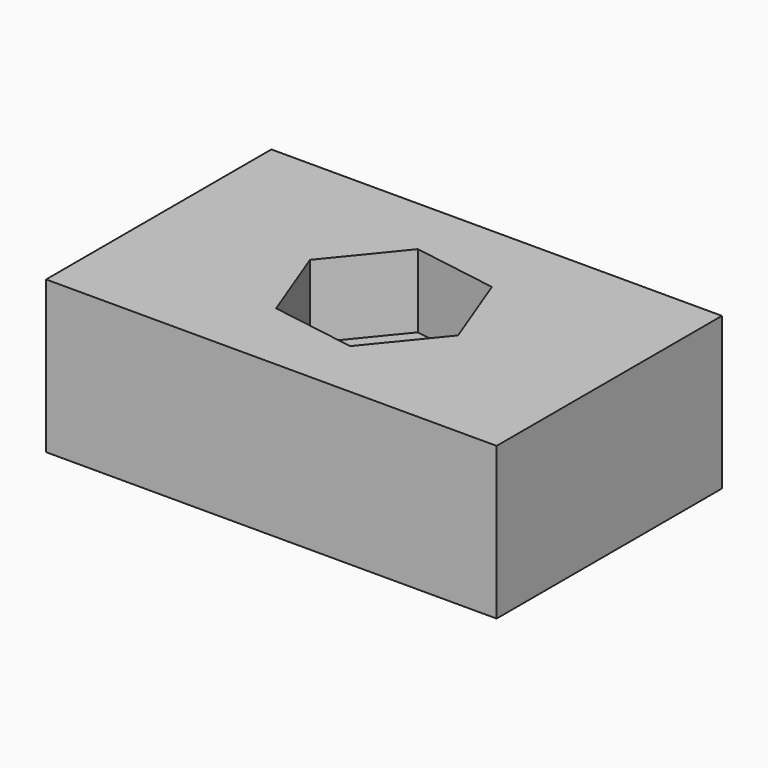
from build123d import *

# Parameters (mm, degrees)
F0_W     = 40
F0_H     = 25
F1_DEPTH = 7
F3_DEPTH = 6.5
F4_R     = 4.75
F5_DEPTH = 10


# Not quite as in the source:
# - a feature names something its author has since deleted; it is built from what else it names


with BuildPart() as f1:
    # F0 (on Top) → F1 (new body)
    with BuildSketch(Plane.XY):
        Rectangle(F0_W, F0_H)
        Polygon((-2.7157951384, 7.1515935357), (4.8355641102, 5.9277443492), (7.5513592486, -1.2238491865), (2.7157951384, -7.1515935357), (-4.8355641102, -5.9277443492), (-7.5513592486, 1.2238491865), align=None, mode=Mode.SUBTRACT)
        Polygon((7.5513592486, -1.2238491865), (4.8355641102, 5.9277443492), (-2.7157951384, 7.1515935357), (-7.5513592486, 1.2238491865), (-4.8355641102, -5.9277443492), (2.7157951384, -7.1515935357), align=None)
    extrude(amount=-F1_DEPTH)

    # F0 (on Top) → F3 (join)
    with BuildSketch(Plane.XY):
        Rectangle(F0_W, F0_H)
        Polygon((-2.7157951384, 7.1515935357), (4.8355641102, 5.9277443492), (7.5513592486, -1.2238491865), (2.7157951384, -7.1515935357), (-4.8355641102, -5.9277443492), (-7.5513592486, 1.2238491865), align=None, mode=Mode.SUBTRACT)
    extrude(amount=F3_DEPTH)

    # F4 (on Top) → F5 (cut)
    with BuildSketch(Plane.XY):
        Circle(F4_R)
    extrude(amount=-F5_DEPTH, mode=Mode.SUBTRACT)


solid = f1.part
